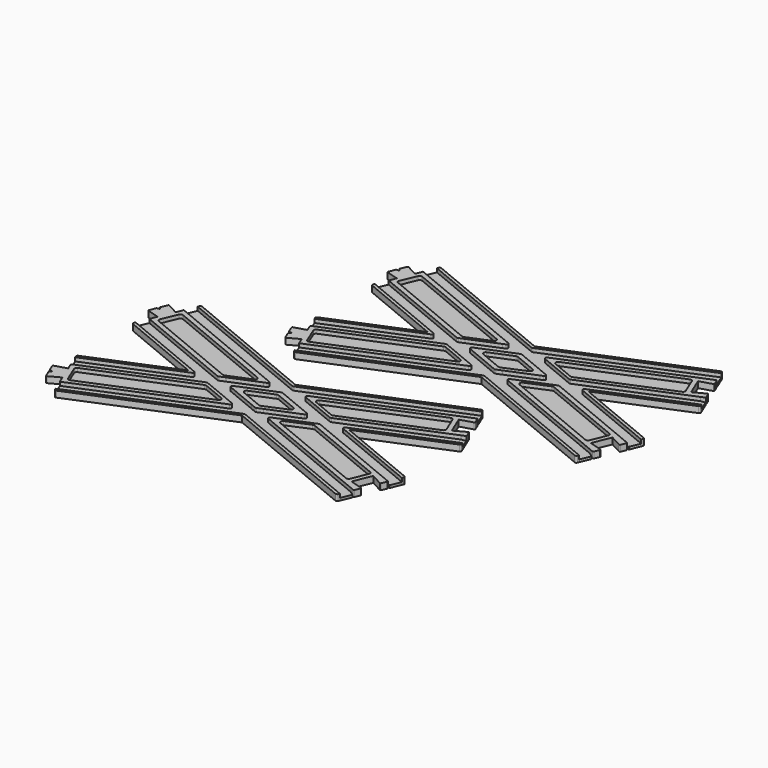
from build123d import *

# Parameters (mm, degrees)
F1_DEPTH = 0.8
F2_DEPTH = 2


# Not quite as in the source:
# - a feature names something its author has since deleted; it is built from what else it names


with BuildPart() as f1:
    # F0 (on Top) → F1 (new body)
    with BuildSketch(Plane.XY):
        with BuildLine():
            Line((-26.799640073, -15.3443313502), (-63.0164195978, -0.3428500855))
            ThreePointArc((-63.0164195978, -0.3428500855), (-63.5904447463, -0.3428500855), (-63.9963418214, -0.7487471607))
            Line((-63.9963418214, -0.7487471607), (-66.1011006995, -5.8300845895))
            ThreePointArc((-66.1011006995, -5.8300845895), (-66.1011006995, -6.404109738), (-65.6952036243, -6.8100068131))
            Line((-65.6952036243, -6.8100068131), (-34.6554323865, -19.6671010328))
            ThreePointArc((-34.6554323865, -19.6671010328), (-34.2727489541, -19.7432215003), (-33.8900655217, -19.6671010328))
            Line((-33.8900655217, -19.6671010328), (-26.799640073, -16.730150649))
            ThreePointArc((-26.799640073, -16.730150649), (-26.3366526473, -16.0372409996), (-26.799640073, -15.3443313502))
        make_face()
    extrude(amount=F1_DEPTH)


with BuildPart() as f1b:
    # F0 (on Top) → F1, piece 2 (new body)
    with BuildSketch(Plane.XY):
        with BuildLine():
            Line((-41.3631744028, -23.7656999509), (-69.878690808, -35.577213584))
            Line((-69.878690808, -35.577213584), (-68.3479570786, -39.272731714))
            Line((-68.3479570786, -39.272731714), (-35.3087138689, -25.587429086))
            ThreePointArc((-35.3087138689, -25.587429086), (-35.0217012946, -25.5303387354), (-34.7346887203, -25.587429086))
            Line((-34.7346887203, -25.587429086), (-23.0712928945, -30.4185658204))
            ThreePointArc((-23.0712928945, -30.4185658204), (-22.7626346107, -30.8805055866), (-23.0712928945, -31.3424453529))
            Line((-23.0712928945, -31.3424453529), (-64.5211227549, -48.5115270391))
            Line((-64.5211227549, -48.5115270391), (-62.9903890255, -52.2070451692))
            Line((-62.9903890255, -52.2070451692), (-17.0168323606, -33.1641744881))
            ThreePointArc((-17.0168323606, -33.1641744881), (-16.7298197863, -33.1070841375), (-16.4428072121, -33.1641744881))
            Line((-16.4428072121, -33.1641744881), (29.5314184974, -52.2073222965))
            Line((29.5314184974, -52.2073222965), (30.9090788598, -48.8813559653))
            Line((30.9090788598, -48.8813559653), (29.6756608657, -47.9375006406))
            Line((29.6756608657, -47.9375006406), (-10.3883466781, -31.3424453529))
            ThreePointArc((-10.3883466781, -31.3424453529), (-10.697004962, -30.8805055866), (-10.3883466781, -30.4185658204))
            Line((-10.3883466781, -30.4185658204), (-9.5437234795, -30.0687114364))
            Line((-9.5437234795, -30.0687114364), (-0.3977827254, -26.2803387354))
            Line((-0.3977827254, -26.2803387354), (1.2750493395, -25.5874290065))
            ThreePointArc((1.2750493395, -25.5874290065), (1.5620619138, -25.5303386559), (1.8490744881, -25.5874290065))
            Line((1.8490744881, -25.5874290065), (33.5024952456, -38.6987051798))
            Line((33.5024952456, -38.6987051798), (35.0420599293, -38.9034570142))
            Line((35.0420599293, -38.9034570142), (36.4197203362, -35.5774905756))
            Line((36.4197203362, -35.5774905756), (7.903535022, -23.7656998714))
            ThreePointArc((7.903535022, -23.7656998714), (7.5948767382, -23.3037601051), (7.903535022, -22.8418203389))
            Line((7.903535022, -22.8418203389), (36.4190482408, -11.0303080256))
            Line((36.4190482408, -11.0303080256), (35.0413878843, -7.7043417086))
            Line((35.0413878843, -7.7043417086), (33.5024956723, -7.9088148537))
            Line((33.5024956723, -7.9088148537), (1.8490744881, -21.0200912037))
            ThreePointArc((1.8490744881, -21.0200912037), (1.5620619138, -21.0771815543), (1.2750493395, -21.0200912037))
            Line((1.2750493395, -21.0200912037), (-10.3883464863, -16.1889544693))
            ThreePointArc((-10.3883464863, -16.1889544693), (-10.6970047701, -15.7270147031), (-10.3883464863, -15.2650749368))
            Line((-10.3883464863, -15.2650749368), (29.6756612258, 1.3299804205))
            Line((29.6756612258, 1.3299804205), (30.9084068147, 2.2735572425))
            Line((30.9084068147, 2.2735572425), (29.5307464582, 5.5995235596))
            Line((29.5307464582, 5.5995235596), (-16.4428070202, -13.4433458017))
            ThreePointArc((-16.4428070202, -13.4433458017), (-16.7298195945, -13.5004361523), (-17.0168321687, -13.4433458017))
            Line((-17.0168321687, -13.4433458017), (-62.9903896117, 5.5995252018))
            Line((-62.9903896117, 5.5995252018), (-64.5211233412, 1.9040070717))
            Line((-64.5211233412, 1.9040070717), (-23.0712927027, -15.2650749368))
            ThreePointArc((-23.0712927027, -15.2650749368), (-22.7626344189, -15.7270147031), (-23.0712927027, -16.1889544693))
            Line((-23.0712927027, -16.1889544693), (-23.9159160932, -16.5388089328))
            Line((-23.9159160932, -16.5388089328), (-33.0618568473, -20.3271816338))
            Line((-33.0618568473, -20.3271816338), (-34.7346887203, -21.0200912832))
            ThreePointArc((-34.7346887203, -21.0200912832), (-35.0217012946, -21.0771816338), (-35.3087138689, -21.0200912832))
            Line((-35.3087138689, -21.0200912832), (-68.347957721, -7.3347883891))
            Line((-68.347957721, -7.3347883891), (-69.8786914505, -11.0303065191))
            Line((-69.8786914505, -11.0303065191), (-41.3631744028, -22.8418204183))
            ThreePointArc((-41.3631744028, -22.8418204183), (-41.054516119, -23.3037601846), (-41.3631744028, -23.7656999509))
        make_face()
        with BuildLine():
            Line((-18.6432387783, -27.9231570891), (-28.6802281864, -23.7656999509))
            ThreePointArc((-28.6802281864, -23.7656999509), (-28.9888864702, -23.3037601846), (-28.6802281864, -22.8418204183))
            Line((-28.6802281864, -22.8418204183), (-27.8356049878, -22.4919660344))
            Line((-27.8356049878, -22.4919660344), (-18.6896642337, -18.7035933334))
            Line((-18.6896642337, -18.7035933334), (-18.6432384455, -18.6843631422))
            Line((-18.6432384455, -18.6843631422), (-17.0168321687, -18.0106836045))
            ThreePointArc((-17.0168321687, -18.0106836045), (-16.7298195945, -17.9535932539), (-16.4428070202, -18.0106836045))
            Line((-16.4428070202, -18.0106836045), (-14.8164043984, -18.6843616283))
            Line((-14.8164043984, -18.6843616283), (-14.7699751472, -18.7035932539))
            Line((-14.7699751472, -18.7035932539), (-4.7794111944, -22.8418203389))
            ThreePointArc((-4.7794111944, -22.8418203389), (-4.4707529106, -23.3037601051), (-4.7794111944, -23.7656998714))
            Line((-4.7794111944, -23.7656998714), (-5.6240345849, -24.1155543348))
            Line((-5.6240345849, -24.1155543348), (-14.769975339, -27.9039270358))
            Line((-14.769975339, -27.9039270358), (-16.4428072121, -28.5968366852))
            ThreePointArc((-16.4428072121, -28.5968366852), (-16.7298197863, -28.6539270358), (-17.0168323606, -28.5968366852))
            Line((-17.0168323606, -28.5968366852), (-18.6432387783, -27.9231570891))
        make_face(mode=Mode.SUBTRACT)
    extrude(amount=F1_DEPTH)


with BuildPart() as f1c:
    # F0 (on Top) → F1, piece 3 (new body)
    with BuildSketch(Plane.XY):
        with BuildLine():
            Line((-34.7511032445, -26.9800475033), (-65.6952029819, -39.79751329))
            ThreePointArc((-65.6952029819, -39.79751329), (-66.101100057, -40.2034103651), (-66.101100057, -40.7774355136))
            Line((-66.101100057, -40.7774355136), (-63.996341179, -45.8587729424))
            ThreePointArc((-63.996341179, -45.8587729424), (-63.5904441039, -46.2646700175), (-63.0164189553, -46.2646700175))
            Line((-63.0164189553, -46.2646700175), (-26.8953109311, -31.302817186))
            ThreePointArc((-26.8953109311, -31.302817186), (-26.4323235054, -30.6099075366), (-26.8953109311, -29.9169978872))
            Line((-26.8953109311, -29.9169978872), (-33.9857363798, -26.9800475033))
            ThreePointArc((-33.9857363798, -26.9800475033), (-34.3684198122, -26.9039270358), (-34.7511032445, -26.9800475033))
        make_face()
    extrude(amount=F1_DEPTH)


with BuildPart() as f1d:
    # F0 (on Top) → F1, piece 4 (new body)
    with BuildSketch(Plane.XY):
        with BuildLine():
            ThreePointArc((-24.2029286674, -22.6108505352), (-24.6659160932, -23.3037601846), (-24.2029286674, -23.996669834))
            Line((-24.2029286674, -23.996669834), (-17.0168323606, -26.9732483848))
            ThreePointArc((-17.0168323606, -26.9732483848), (-16.629331896, -27.0493572503), (-16.2425826435, -26.9695187556))
            Line((-16.2425826435, -26.9695187556), (-9.250048766, -23.9938726121))
            ThreePointArc((-9.250048766, -23.9938726121), (-8.793732181, -23.3001474104), (-9.2567109053, -22.6108505352))
            Line((-9.2567109053, -22.6108505352), (-16.347136354, -19.6739001514))
            ThreePointArc((-16.347136354, -19.6739001514), (-16.7298197863, -19.5977796839), (-17.1125032187, -19.6739001514))
            Line((-17.1125032187, -19.6739001514), (-24.2029286674, -22.6108505352))
        make_face()
    extrude(amount=F1_DEPTH)


with BuildPart() as f1e:
    # F0 (on Top) → F1, piece 5 (new body)
    with BuildSketch(Plane.XY):
        with BuildLine():
            Line((28.532860387, -7.6111790722), (26.4000801634, -2.4621921308))
            ThreePointArc((26.4000801634, -2.4621921308), (25.9941830883, -2.0562950557), (25.4201579397, -2.0562950557))
            Line((25.4201579397, -2.0562950557), (-6.5643284497, -15.3047031038))
            ThreePointArc((-6.5643284497, -15.3047031038), (-7.0273158755, -15.9976127532), (-6.5643284497, -16.6905224025))
            Line((-6.5643284497, -16.6905224025), (0.6217678571, -19.6671009533))
            ThreePointArc((0.6217678571, -19.6671009533), (1.0044512894, -19.7432214208), (1.3871347218, -19.6671009533))
            Line((1.3871347218, -19.6671009533), (28.1269633119, -8.5911012958))
            ThreePointArc((28.1269633119, -8.5911012958), (28.532860387, -8.1852042207), (28.532860387, -7.6111790722))
        make_face()
    extrude(amount=F1_DEPTH)


with BuildPart() as f1f:
    # F0 (on Top) → F1, piece 6 (new body)
    with BuildSketch(Plane.XY):
        with BuildLine():
            Line((26.4000800865, -44.1453282065), (28.5048389645, -39.0639907777))
            ThreePointArc((28.5048389645, -39.0639907777), (28.5048389645, -38.4899656292), (28.0989418894, -38.0840685541))
            Line((28.0989418894, -38.0840685541), (1.1957928138, -26.9404193364))
            ThreePointArc((1.1957928138, -26.9404193364), (0.8082923491, -26.8643104709), (0.4215430966, -26.9441489655))
            Line((0.4215430966, -26.9441489655), (-6.5709907809, -29.9197951091))
            ThreePointArc((-6.5709907809, -29.9197951091), (-7.0273073659, -30.6135203108), (-6.5643286416, -31.302817186))
            Line((-6.5643286416, -31.302817186), (25.4201578629, -44.5512252817))
            ThreePointArc((25.4201578629, -44.5512252817), (25.9941830114, -44.5512252817), (26.4000800865, -44.1453282065))
        make_face()
    extrude(amount=F1_DEPTH)


with BuildPart() as f1g:
    # F0 (on Top) → F1, piece 7 (new body)
    with BuildSketch(Plane.XY):
        with BuildLine():
            Line((-7.114914129, 30.7077025481), (-35.6304305342, 18.896188915))
            Line((-35.6304305342, 18.896188915), (-34.0996968047, 15.200670785))
            Line((-34.0996968047, 15.200670785), (-1.060453595, 28.885973413))
            ThreePointArc((-1.060453595, 28.885973413), (-0.7734410208, 28.9430637636), (-0.4864284465, 28.885973413))
            Line((-0.4864284465, 28.885973413), (11.1769673793, 24.0548366786))
            ThreePointArc((11.1769673793, 24.0548366786), (11.4856256631, 23.5928969123), (11.1769673793, 23.1309571461))
            Line((11.1769673793, 23.1309571461), (-30.2728624811, 5.9618754599))
            Line((-30.2728624811, 5.9618754598), (-28.7421287516, 2.2663573298))
            Line((-28.7421287516, 2.2663573298), (17.2314279132, 21.3092280109))
            ThreePointArc((17.2314279132, 21.3092280109), (17.5184404875, 21.3663183615), (17.8054530618, 21.3092280109))
            Line((17.8054530618, 21.3092280109), (63.7796787572, 2.2660802083))
            Line((63.7796787572, 2.2660802083), (65.1573391196, 5.5920465395))
            Line((65.1573391196, 5.5920465395), (63.9239211396, 6.5359018584))
            Line((63.9239211396, 6.5359018584), (23.8599135957, 23.1309571461))
            ThreePointArc((23.8599135957, 23.1309571461), (23.5512553119, 23.5928969123), (23.8599135957, 24.0548366786))
            Line((23.8599135957, 24.0548366786), (24.7045367943, 24.4046910626))
            Line((24.7045367943, 24.4046910626), (33.8504775485, 28.1930637636))
            Line((33.8504775485, 28.1930637636), (35.5233096134, 28.8859734924))
            ThreePointArc((35.5233096134, 28.8859734924), (35.8103221876, 28.9430638431), (36.0973347619, 28.8859734924))
            Line((36.0973347619, 28.8859734924), (67.7507555194, 15.7746973192))
            Line((67.7507555194, 15.7746973192), (69.2903201891, 15.5699454906))
            Line((69.2903201891, 15.5699454906), (70.667980596, 18.8959119292))
            Line((70.667980596, 18.8959119292), (42.1517952958, 30.7077026276))
            ThreePointArc((42.1517952958, 30.7077026276), (41.843137012, 31.1696423939), (42.1517952958, 31.6315821601))
            Line((42.1517952958, 31.6315821601), (70.6673085146, 43.4430944734))
            Line((70.6673085146, 43.4430944734), (69.2896481581, 46.7690607904))
            Line((69.2896481581, 46.7690607904), (67.7507559462, 46.5645876453))
            Line((67.7507559462, 46.5645876453), (36.0973347619, 33.4533112953))
            ThreePointArc((36.0973347619, 33.4533112953), (35.8103221876, 33.3962209447), (35.5233096134, 33.4533112953))
            Line((35.5233096134, 33.4533112953), (23.8599137876, 38.2844480297))
            ThreePointArc((23.8599137876, 38.2844480297), (23.5512555037, 38.7463877959), (23.8599137876, 39.2083275622))
            Line((23.8599137876, 39.2083275622), (63.9239214996, 55.8033829195))
            Line((63.9239214996, 55.8033829195), (65.1566670886, 56.7469597415))
            Line((65.1566670886, 56.7469597415), (63.7790067321, 60.0729260586))
            Line((63.7790067321, 60.0729260586), (17.8054532536, 41.0300566973))
            ThreePointArc((17.8054532536, 41.0300566973), (17.5184406794, 40.9729663467), (17.2314281051, 41.0300566973))
            Line((17.2314281051, 41.0300566973), (-28.7421293379, 60.0729277008))
            Line((-28.7421293379, 60.0729277008), (-30.2728630674, 56.3774095707))
            Line((-30.2728630674, 56.3774095707), (11.1769675712, 39.2083275622))
            ThreePointArc((11.1769675712, 39.2083275622), (11.485625855, 38.7463877959), (11.1769675712, 38.2844480297))
            Line((11.1769675712, 38.2844480297), (10.3323441807, 37.9345935662))
            Line((10.3323441807, 37.9345935662), (1.1864034265, 34.1462208652))
            Line((1.1864034265, 34.1462208652), (-0.4864284465, 33.4533112158))
            ThreePointArc((-0.4864284465, 33.4533112158), (-0.7734410208, 33.3962208652), (-1.060453595, 33.4533112158))
            Line((-1.060453595, 33.4533112158), (-34.0996974472, 47.1386141099))
            Line((-34.0996974472, 47.1386141099), (-35.6304311767, 43.4430959799))
            Line((-35.6304311767, 43.4430959799), (-7.114914129, 31.6315820806))
            ThreePointArc((-7.114914129, 31.6315820806), (-6.8062558452, 31.1696423144), (-7.114914129, 30.7077025481))
        make_face()
        with BuildLine():
            Line((15.6050214956, 26.5502454099), (5.5680320874, 30.7077025481))
            ThreePointArc((5.5680320874, 30.7077025481), (5.2593738036, 31.1696423144), (5.5680320874, 31.6315820806))
            Line((5.5680320874, 31.6315820806), (6.412655286, 31.9814364646))
            Line((6.412655286, 31.9814364646), (15.5585960402, 35.7698091656))
            Line((15.5585960402, 35.7698091656), (15.6050218284, 35.7890393567))
            Line((15.6050218284, 35.7890393567), (17.2314281051, 36.4627188945))
            ThreePointArc((17.2314281051, 36.4627188945), (17.5184406794, 36.5198092451), (17.8054532536, 36.4627188945))
            Line((17.8054532536, 36.4627188945), (19.4318558754, 35.7890408707))
            Line((19.4318558754, 35.7890408707), (19.4782851267, 35.7698092451))
            Line((19.4782851267, 35.7698092451), (29.4688490794, 31.6315821601))
            ThreePointArc((29.4688490794, 31.6315821601), (29.7775073633, 31.1696423939), (29.4688490794, 30.7077026276))
            Line((29.4688490794, 30.7077026276), (28.6242256889, 30.3578481642))
            Line((28.6242256889, 30.3578481642), (19.4782849348, 26.5694754631))
            Line((19.4782849348, 26.5694754631), (17.8054530618, 25.8765658138))
            ThreePointArc((17.8054530618, 25.8765658138), (17.5184404875, 25.8194754631), (17.2314279132, 25.8765658138))
            Line((17.2314279132, 25.8765658138), (15.6050214956, 26.5502454099))
        make_face(mode=Mode.SUBTRACT)
    extrude(amount=F1_DEPTH)


with BuildPart() as f1h:
    # F0 (on Top) → F1, piece 8 (new body)
    with BuildSketch(Plane.XY):
        with BuildLine():
            Line((7.4486202008, 39.1290711488), (-28.768159324, 54.1305524134))
            ThreePointArc((-28.768159324, 54.1305524134), (-29.3421844725, 54.1305524134), (-29.7480815476, 53.7246553383))
            Line((-29.7480815476, 53.7246553383), (-31.8528404256, 48.6433179095))
            ThreePointArc((-31.8528404256, 48.6433179095), (-31.8528404256, 48.069292761), (-31.4469433505, 47.6633956859))
            Line((-31.4469433505, 47.6633956859), (-0.4071721126, 34.8063014662))
            ThreePointArc((-0.4071721126, 34.8063014662), (-0.0244886802, 34.7301809987), (0.3581947521, 34.8063014662))
            Line((0.3581947521, 34.8063014662), (7.4486202008, 37.74325185))
            ThreePointArc((7.4486202008, 37.74325185), (7.9116076266, 38.4361614994), (7.4486202008, 39.1290711488))
        make_face()
    extrude(amount=F1_DEPTH)


with BuildPart() as f1i:
    # F0 (on Top) → F1, piece 9 (new body)
    with BuildSketch(Plane.XY):
        with BuildLine():
            ThreePointArc((10.0453316064, 31.8625519638), (9.5823441807, 31.1696423144), (10.0453316064, 30.476732665))
            Line((10.0453316064, 30.476732665), (17.2314279132, 27.5001541142))
            ThreePointArc((17.2314279132, 27.5001541142), (17.6189283779, 27.4240452487), (18.0056776303, 27.5038837433))
            Line((18.0056776303, 27.5038837433), (24.9982115079, 30.4795298869))
            ThreePointArc((24.9982115079, 30.4795298869), (25.4545280928, 31.1732550886), (24.9915493686, 31.8625519638))
            Line((24.9915493686, 31.8625519638), (17.9011239199, 34.7995023476))
            ThreePointArc((17.9011239199, 34.7995023476), (17.5184404875, 34.8756228151), (17.1357570551, 34.7995023476))
            Line((17.1357570551, 34.7995023476), (10.0453316064, 31.8625519638))
        make_face()
    extrude(amount=F1_DEPTH)


with BuildPart() as f1j:
    # F0 (on Top) → F1, piece 10 (new body)
    with BuildSketch(Plane.XY):
        with BuildLine():
            Line((62.7811206608, 46.8622234268), (60.6483404372, 52.0112103682))
            ThreePointArc((60.6483404372, 52.0112103682), (60.2424433621, 52.4171074433), (59.6684182136, 52.4171074433))
            Line((59.6684182136, 52.4171074433), (27.6839318241, 39.1686993952))
            ThreePointArc((27.6839318241, 39.1686993952), (27.2209443984, 38.4757897458), (27.6839318241, 37.7828800964))
            Line((27.6839318241, 37.7828800964), (34.8700281309, 34.8063015456))
            ThreePointArc((34.8700281309, 34.8063015456), (35.2527115633, 34.7301810782), (35.6353949957, 34.8063015456))
            Line((35.6353949957, 34.8063015456), (62.3752235857, 45.8823012032))
            ThreePointArc((62.3752235857, 45.8823012032), (62.7811206608, 46.2881982783), (62.7811206608, 46.8622234268))
        make_face()
    extrude(amount=F1_DEPTH)


with BuildPart() as f1k:
    # F0 (on Top) → F1, piece 11 (new body)
    with BuildSketch(Plane.XY):
        with BuildLine():
            Line((60.6483403619, 10.3280742918), (62.7530992399, 15.4094117206))
            ThreePointArc((62.7530992399, 15.4094117206), (62.7530992399, 15.9834368692), (62.3472021648, 16.3893339443))
            Line((62.3472021648, 16.3893339443), (35.4440530876, 27.5329831626))
            ThreePointArc((35.4440530876, 27.5329831626), (35.0565526229, 27.6090920281), (34.6698033705, 27.5292535334))
            Line((34.6698033705, 27.5292535334), (27.6772694929, 24.5536073899))
            ThreePointArc((27.6772694929, 24.5536073899), (27.220952908, 23.8598821882), (27.6839316322, 23.170585313))
            Line((27.6839316322, 23.170585313), (59.6684181383, 9.9221772167))
            ThreePointArc((59.6684181383, 9.9221772167), (60.2424432868, 9.9221772167), (60.6483403619, 10.3280742918))
        make_face()
    extrude(amount=F1_DEPTH)


with BuildPart() as f1l:
    # F0 (on Top) → F1, piece 12 (new body)
    with BuildSketch(Plane.XY):
        with BuildLine():
            Line((-0.5028429707, 27.4933549957), (-31.446942708, 14.675889209))
            ThreePointArc((-31.446942708, 14.675889209), (-31.8528397832, 14.2699921339), (-31.8528397832, 13.6959669854))
            Line((-31.8528397832, 13.6959669854), (-29.7480809051, 8.6146295565))
            ThreePointArc((-29.7480809051, 8.6146295565), (-29.34218383, 8.2087324814), (-28.7681586815, 8.2087324814))
            Line((-28.7681586815, 8.2087324814), (7.3529493428, 23.170585313))
            ThreePointArc((7.3529493428, 23.170585313), (7.8159367685, 23.8634949624), (7.3529493428, 24.5564046118))
            Line((7.3529493428, 24.5564046118), (0.262523894, 27.4933549957))
            ThreePointArc((0.262523894, 27.4933549957), (-0.1201595383, 27.5694754631), (-0.5028429707, 27.4933549957))
        make_face()
    extrude(amount=F1_DEPTH)


with BuildPart() as f2:
    # F0 (on Top) → F2 (new body)
    with BuildSketch(Plane.XY):
        with BuildLine():
            Line((-67.4295174834, -5.117477511), (-68.347957721, -7.3347883891))
            Line((-68.347957721, -7.3347883891), (-35.3087138689, -21.0200912832))
            ThreePointArc((-35.3087138689, -21.0200912832), (-35.0217012946, -21.0771816338), (-34.7346887203, -21.0200912832))
            Line((-34.7346887203, -21.0200912832), (-33.0618568473, -20.3271816338))
            Line((-33.0618568473, -20.3271816338), (-23.9159160932, -16.5388089328))
            Line((-23.9159160932, -16.5388089328), (-23.0712927027, -16.1889544693))
            ThreePointArc((-23.0712927027, -16.1889544693), (-22.7626344189, -15.7270147031), (-23.0712927027, -15.2650749368))
            Line((-23.0712927027, -15.2650749368), (-64.5211233412, 1.9040070717))
            Line((-64.5211233412, 1.9040070717), (-65.4395635789, -0.3133038063))
            Line((-65.4395635789, -0.3133038063), (-68.9742038238, 1.6064137918))
            ThreePointArc((-68.9742038238, 1.6064137918), (-69.1769577929, 1.6223897475), (-69.3244904948, 1.4823950868))
            Line((-69.3244904948, 1.4823950868), (-70.1940668164, -0.6169478625))
            Line((-70.1940668164, -0.6169478625), (-69.5853053874, -1.4103012028))
            Line((-69.5853053874, -1.4103012028), (-70.5767502345, -1.5408274009))
            Line((-70.5767502345, -1.5408274009), (-71.4463265525, -3.6401703414))
            ThreePointArc((-71.4463265525, -3.6401703414), (-71.4409963507, -3.8434828932), (-71.2863309312, -3.9755548915))
            Line((-71.2863309312, -3.9755548915), (-67.4295174834, -5.117477511))
        make_face()
        with BuildLine():
            ThreePointArc((-63.9963418214, -0.7487471607), (-63.5904447463, -0.3428500855), (-63.0164195978, -0.3428500855))
            Line((-63.0164195978, -0.3428500855), (-26.799640073, -15.3443313502))
            ThreePointArc((-26.799640073, -15.3443313502), (-26.3366526473, -16.0372409996), (-26.799640073, -16.730150649))
            Line((-26.799640073, -16.730150649), (-33.8900655217, -19.6671010328))
            ThreePointArc((-33.8900655217, -19.6671010328), (-34.2727489541, -19.7432215003), (-34.6554323865, -19.6671010328))
            Line((-34.6554323865, -19.6671010328), (-65.6952036243, -6.8100068131))
            ThreePointArc((-65.6952036243, -6.8100068131), (-66.1011006995, -6.404109738), (-66.1011006995, -5.8300845895))
            Line((-66.1011006995, -5.8300845895), (-63.9963418214, -0.7487471607))
        make_face(mode=Mode.SUBTRACT)
    extrude(amount=F2_DEPTH)


with BuildPart() as f2b:
    # F0 (on Top) → F2, piece 2 (new body)
    with BuildSketch(Plane.XY):
        with BuildLine():
            Line((-42.8610790839, -23.3037601846), (-69.7994344742, -34.4619923353))
            ThreePointArc((-69.7994344742, -34.4619923353), (-70.0700325242, -34.7325903854), (-70.0700325242, -35.1152738177))
            Line((-70.0700325242, -35.1152738177), (-69.878690808, -35.577213584))
            Line((-69.878690808, -35.577213584), (-41.3631744028, -23.7656999509))
            ThreePointArc((-41.3631744028, -23.7656999509), (-41.054516119, -23.3037601846), (-41.3631744028, -22.8418204183))
            Line((-41.3631744028, -22.8418204183), (-69.8786914505, -11.0303065191))
            Line((-69.8786914505, -11.0303065191), (-70.0700331667, -11.4922462854))
            ThreePointArc((-70.0700331667, -11.4922462854), (-70.0700331667, -11.8749297177), (-69.7994351166, -12.1455277678))
            Line((-69.7994351166, -12.1455277678), (-42.8610790839, -23.3037601846))
        make_face()
    extrude(amount=F2_DEPTH)


with BuildPart() as f2c:
    # F0 (on Top) → F2, piece 3 (new body)
    with BuildSketch(Plane.XY):
        with BuildLine():
            Line((-35.3087138689, -25.587429086), (-68.3479570786, -39.272731714))
            Line((-68.3479570786, -39.272731714), (-67.4295168409, -41.490042592))
            Line((-67.4295168409, -41.490042592), (-71.2863302887, -42.6319652115))
            ThreePointArc((-71.2863302887, -42.6319652115), (-71.4409957082, -42.7640372099), (-71.4463259101, -42.9673497617))
            Line((-71.4463259101, -42.9673497617), (-70.5767495921, -45.0666927021))
            Line((-70.5767495921, -45.0666927021), (-69.5853047307, -45.1972188944))
            Line((-69.5853047307, -45.1972188944), (-70.1940661597, -45.9905722347))
            Line((-70.1940661597, -45.9905722347), (-69.3244898417, -48.0899151751))
            ThreePointArc((-69.3244898417, -48.0899151751), (-69.1769571358, -48.2299098373), (-68.9742031631, -48.213933876))
            Line((-68.9742031631, -48.213933876), (-65.4395629926, -46.2942161611))
            Line((-65.4395629926, -46.2942161611), (-64.5211227549, -48.5115270391))
            Line((-64.5211227549, -48.5115270391), (-23.0712928945, -31.3424453529))
            ThreePointArc((-23.0712928945, -31.3424453529), (-22.7626346107, -30.8805055866), (-23.0712928945, -30.4185658204))
            Line((-23.0712928945, -30.4185658204), (-34.7346887203, -25.587429086))
            ThreePointArc((-34.7346887203, -25.587429086), (-35.0217012946, -25.5303387354), (-35.3087138689, -25.587429086))
        make_face()
        with BuildLine():
            ThreePointArc((-66.101100057, -40.7774355136), (-66.101100057, -40.2034103651), (-65.6952029819, -39.79751329))
            Line((-65.6952029819, -39.79751329), (-34.7511032445, -26.9800475033))
            ThreePointArc((-34.7511032445, -26.9800475033), (-34.3684198122, -26.9039270358), (-33.9857363798, -26.9800475033))
            Line((-33.9857363798, -26.9800475033), (-26.8953109311, -29.9169978872))
            ThreePointArc((-26.8953109311, -29.9169978872), (-26.4323235054, -30.6099075366), (-26.8953109311, -31.302817186))
            Line((-26.8953109311, -31.302817186), (-63.0164189553, -46.2646700175))
            ThreePointArc((-63.0164189553, -46.2646700175), (-63.5904441039, -46.2646700175), (-63.996341179, -45.8587729424))
            Line((-63.996341179, -45.8587729424), (-66.101100057, -40.7774355136))
        make_face(mode=Mode.SUBTRACT)
    extrude(amount=F2_DEPTH)


with BuildPart() as f2d:
    # F0 (on Top) → F2, piece 4 (new body)
    with BuildSketch(Plane.XY):
        with BuildLine():
            Line((-17.0168323606, -33.1641744881), (-62.9903890255, -52.2070451692))
            Line((-62.9903890255, -52.2070451692), (-62.7990473093, -52.6689849354))
            ThreePointArc((-62.7990473093, -52.6689849354), (-62.5284492592, -52.9395829855), (-62.1457658269, -52.9395829855))
            Line((-62.1457658269, -52.9395829855), (-16.7298197863, -34.1276821875))
            Line((-16.7298197863, -34.1276821875), (28.6867952988, -52.9398601129))
            ThreePointArc((28.6867952988, -52.9398601129), (29.0694787311, -52.9398601129), (29.3400767812, -52.6692620628))
            Line((29.3400767812, -52.6692620628), (29.5314184974, -52.2073222965))
            Line((29.5314184974, -52.2073222965), (-16.4428072121, -33.1641744881))
            ThreePointArc((-16.4428072121, -33.1641744881), (-16.7298197863, -33.1070841375), (-17.0168323606, -33.1641744881))
        make_face()
    extrude(amount=F2_DEPTH)


with BuildPart() as f2e:
    # F0 (on Top) → F2, piece 5 (new body)
    with BuildSketch(Plane.XY):
        with BuildLine():
            Line((-10.3883466781, -31.3424453529), (29.6756608657, -47.9375006406))
            Line((29.6756608657, -47.9375006406), (30.8311092685, -48.4161030396))
            ThreePointArc((30.8311092685, -48.4161030396), (31.0224875153, -48.4160879048), (31.1577802621, -48.2807309461))
            Line((31.1577802621, -48.2807309461), (31.8359982031, -46.6419018804))
            ThreePointArc((31.8359982031, -46.6419018804), (31.8308718378, -46.4391544761), (31.6770923803, -46.3069248726))
            Line((31.6770923803, -46.3069248726), (27.6328260153, -45.0889051693))
            Line((27.6328260153, -45.0889051693), (30.0437317475, -39.2684640004))
            Line((30.0437317475, -39.2684640004), (33.764729932, -41.2669221325))
            ThreePointArc((33.764729932, -41.2669221325), (33.9669688804, -41.2821601773), (34.1139578305, -41.142420996))
            Line((34.1139578305, -41.142420996), (34.7932124067, -39.5040213753))
            ThreePointArc((34.7932124067, -39.5040213753), (34.7932578074, -39.3126431364), (34.6579436546, -39.1773075814))
            Line((34.6579436546, -39.1773075814), (33.5024952456, -38.6987051798))
            Line((33.5024952456, -38.6987051798), (1.8490744881, -25.5874290065))
            ThreePointArc((1.8490744881, -25.5874290065), (1.5620619138, -25.5303386559), (1.2750493395, -25.5874290065))
            Line((1.2750493395, -25.5874290065), (-0.3977827254, -26.2803387354))
            Line((-0.3977827254, -26.2803387354), (-9.5437234795, -30.0687114364))
            Line((-9.5437234795, -30.0687114364), (-10.3883466781, -30.4185658204))
            ThreePointArc((-10.3883466781, -30.4185658204), (-10.697004962, -30.8805055866), (-10.3883466781, -31.3424453529))
        make_face()
        with BuildLine():
            ThreePointArc((28.0989418894, -38.0840685541), (28.5048389645, -38.4899656292), (28.5048389645, -39.0639907777))
            Line((28.5048389645, -39.0639907777), (26.4000800865, -44.1453282065))
            ThreePointArc((26.4000800865, -44.1453282065), (25.9941830114, -44.5512252817), (25.4201578629, -44.5512252817))
            Line((25.4201578629, -44.5512252817), (-6.5643286416, -31.302817186))
            ThreePointArc((-6.5643286416, -31.302817186), (-7.0273073659, -30.6135203108), (-6.5709907809, -29.9197951091))
            Line((-6.5709907809, -29.9197951091), (0.4215430966, -26.9441489655))
            ThreePointArc((0.4215430966, -26.9441489655), (0.8082923491, -26.8643104709), (1.1957928138, -26.9404193364))
            Line((1.1957928138, -26.9404193364), (28.0989418894, -38.0840685541))
        make_face(mode=Mode.SUBTRACT)
    extrude(amount=F2_DEPTH)


with BuildPart() as f2f:
    # F0 (on Top) → F2, piece 6 (new body)
    with BuildSketch(Plane.XY):
        with BuildLine():
            Line((7.903535022, -23.7656998714), (36.4197203362, -35.5774905756))
            Line((36.4197203362, -35.5774905756), (36.6110620523, -35.1155508094))
            ThreePointArc((36.6110620523, -35.1155508094), (36.6110620523, -34.732867377), (36.3404640023, -34.462269327))
            Line((36.3404640023, -34.462269327), (9.4014397031, -23.3037601051))
            Line((9.4014397031, -23.3037601051), (36.3397919069, -12.1455292743))
            ThreePointArc((36.3397919069, -12.1455292743), (36.610389957, -11.8749312242), (36.610389957, -11.4922477919))
            Line((36.610389957, -11.4922477919), (36.4190482408, -11.0303080256))
            Line((36.4190482408, -11.0303080256), (7.903535022, -22.8418203389))
            ThreePointArc((7.903535022, -22.8418203389), (7.5948767382, -23.3037601051), (7.903535022, -23.7656998714))
        make_face()
    extrude(amount=F2_DEPTH)


with BuildPart() as f2g:
    # F0 (on Top) → F2, piece 7 (new body)
    with BuildSketch(Plane.XY):
        with BuildLine():
            Line((30.8305103573, 1.8083345933), (29.6756612258, 1.3299804205))
            Line((29.6756612258, 1.3299804205), (-10.3883464863, -15.2650749368))
            ThreePointArc((-10.3883464863, -15.2650749368), (-10.6970047701, -15.7270147031), (-10.3883464863, -16.1889544693))
            Line((-10.3883464863, -16.1889544693), (1.2750493395, -21.0200912037))
            ThreePointArc((1.2750493395, -21.0200912037), (1.5620619138, -21.0771815543), (1.8490744881, -21.0200912037))
            Line((1.8490744881, -21.0200912037), (33.5024956723, -7.9088148537))
            Line((33.5024956723, -7.9088148537), (34.8883145113, -7.3347898956))
            Line((34.8883145113, -7.3347898956), (34.1139106964, -5.465213793))
            ThreePointArc((34.1139106964, -5.465213793), (33.9669287134, -5.3254148419), (33.7646525247, -5.3406396088))
            Line((33.7646525247, -5.3406396088), (30.0437317481, -7.3390562096))
            Line((30.0437317481, -7.3390562096), (27.6328266453, -1.5186149389))
            Line((27.6328266453, -1.5186149389), (31.6770088236, -0.3006205752))
            ThreePointArc((31.6770088236, -0.3006205752), (31.8308052373, -0.1683552187), (31.8358843713, 0.0344295534))
            Line((31.8358843713, 0.0344295534), (31.1571510766, 1.673035621))
            ThreePointArc((31.1571510766, 1.673035621), (31.0218520471, 1.8083346042), (30.8305103573, 1.8083345933))
        make_face()
        with BuildLine():
            ThreePointArc((25.4201579397, -2.0562950557), (25.9941830883, -2.0562950557), (26.4000801634, -2.4621921308))
            Line((26.4000801634, -2.4621921308), (28.532860387, -7.6111790722))
            ThreePointArc((28.532860387, -7.6111790722), (28.532860387, -8.1852042207), (28.1269633119, -8.5911012958))
            Line((28.1269633119, -8.5911012958), (1.3871347218, -19.6671009533))
            ThreePointArc((1.3871347218, -19.6671009533), (1.0044512894, -19.7432214208), (0.6217678571, -19.6671009533))
            Line((0.6217678571, -19.6671009533), (-6.5643284497, -16.6905224025))
            ThreePointArc((-6.5643284497, -16.6905224025), (-7.0273158755, -15.9976127532), (-6.5643284497, -15.3047031038))
            Line((-6.5643284497, -15.3047031038), (25.4201579397, -2.0562950557))
        make_face(mode=Mode.SUBTRACT)
    extrude(amount=F2_DEPTH)


with BuildPart() as f2h:
    # F0 (on Top) → F2, piece 8 (new body)
    with BuildSketch(Plane.XY):
        with BuildLine():
            ThreePointArc((-28.6802281864, -22.8418204183), (-28.9888864702, -23.3037601846), (-28.6802281864, -23.7656999509))
            Line((-28.6802281864, -23.7656999509), (-18.6432387783, -27.9231570891))
            Line((-18.6432387783, -27.9231570891), (-17.0168323606, -28.5968366852))
            ThreePointArc((-17.0168323606, -28.5968366852), (-16.7298197863, -28.6539270358), (-16.4428072121, -28.5968366852))
            Line((-16.4428072121, -28.5968366852), (-14.769975339, -27.9039270358))
            Line((-14.769975339, -27.9039270358), (-5.6240345849, -24.1155543348))
            Line((-5.6240345849, -24.1155543348), (-4.7794111944, -23.7656998714))
            ThreePointArc((-4.7794111944, -23.7656998714), (-4.4707529106, -23.3037601051), (-4.7794111944, -22.8418203389))
            Line((-4.7794111944, -22.8418203389), (-14.7699751472, -18.7035932539))
            Line((-14.7699751472, -18.7035932539), (-14.835636024, -18.7307908796))
            Line((-14.835636024, -18.7307908796), (-14.8164043984, -18.6843616283))
            Line((-14.8164043984, -18.6843616283), (-16.4428070202, -18.0106836045))
            ThreePointArc((-16.4428070202, -18.0106836045), (-16.7298195945, -17.9535932539), (-17.0168321687, -18.0106836045))
            Line((-17.0168321687, -18.0106836045), (-18.6432384455, -18.6843631422))
            Line((-18.6432384455, -18.6843631422), (-18.6896642337, -18.7035933334))
            Line((-18.6896642337, -18.7035933334), (-27.8356049878, -22.4919660344))
            Line((-27.8356049878, -22.4919660344), (-28.6802281864, -22.8418204183))
        make_face()
        with BuildLine():
            Line((-17.0168323606, -26.9732483848), (-24.2029286674, -23.996669834))
            ThreePointArc((-24.2029286674, -23.996669834), (-24.6659160932, -23.3037601846), (-24.2029286674, -22.6108505352))
            Line((-24.2029286674, -22.6108505352), (-17.1125032187, -19.6739001514))
            ThreePointArc((-17.1125032187, -19.6739001514), (-16.7298197863, -19.5977796839), (-16.347136354, -19.6739001514))
            Line((-16.347136354, -19.6739001514), (-9.2567109053, -22.6108505352))
            ThreePointArc((-9.2567109053, -22.6108505352), (-8.793732181, -23.3001474104), (-9.250048766, -23.9938726121))
            Line((-9.250048766, -23.9938726121), (-16.2425826435, -26.9695187556))
            ThreePointArc((-16.2425826435, -26.9695187556), (-16.629331896, -27.0493572503), (-17.0168323606, -26.9732483848))
        make_face(mode=Mode.SUBTRACT)
    extrude(amount=F2_DEPTH)


with BuildPart() as f2i:
    # F0 (on Top) → F2, piece 9 (new body)
    with BuildSketch(Plane.XY):
        with BuildLine():
            Line((-62.7990478956, 6.061464968), (-62.9903896117, 5.5995252018))
            Line((-62.9903896117, 5.5995252018), (-17.0168321687, -13.4433458017))
            ThreePointArc((-17.0168321687, -13.4433458017), (-16.7298195945, -13.5004361523), (-16.4428070202, -13.4433458017))
            Line((-16.4428070202, -13.4433458017), (29.5307464582, 5.5995235596))
            Line((29.5307464582, 5.5995235596), (29.339404742, 6.0614633258))
            ThreePointArc((29.339404742, 6.0614633258), (29.068806692, 6.3320613759), (28.6861232596, 6.3320613759))
            Line((28.6861232596, 6.3320613759), (-16.7298195945, -12.4798381022))
            Line((-16.7298195945, -12.4798381022), (-62.1457664131, 6.3320630181))
            ThreePointArc((-62.1457664131, 6.3320630181), (-62.5284498455, 6.3320630181), (-62.7990478956, 6.061464968))
        make_face()
    extrude(amount=F2_DEPTH)


with BuildPart() as f2j:
    # F0 (on Top) → F2, piece 10 (new body)
    with BuildSketch(Plane.XY):
        with BuildLine():
            Line((-1.060453595, 28.885973413), (-34.0996968047, 15.200670785))
            Line((-34.0996968047, 15.200670785), (-33.1812565671, 12.9833599069))
            Line((-33.1812565671, 12.9833599069), (-37.0380700149, 11.8414372874))
            ThreePointArc((-37.0380700149, 11.8414372874), (-37.1927354344, 11.7093652891), (-37.1980656362, 11.5060527373))
            Line((-37.1980656362, 11.5060527373), (-36.3284893182, 9.4067097968))
            Line((-36.3284893182, 9.4067097968), (-35.3370444569, 9.2761836046))
            Line((-35.3370444569, 9.2761836046), (-35.9458058859, 8.4828302643))
            Line((-35.9458058859, 8.4828302643), (-35.0762295679, 6.3834873239))
            ThreePointArc((-35.0762295679, 6.3834873239), (-34.928696862, 6.2434926617), (-34.7259428893, 6.259468623))
            Line((-34.7259428893, 6.259468623), (-31.1913027188, 8.1791863379))
            Line((-31.1913027188, 8.1791863379), (-30.2728624811, 5.9618754599))
            Line((-30.2728624811, 5.9618754599), (11.1769673793, 23.1309571461))
            ThreePointArc((11.1769673793, 23.1309571461), (11.4856256631, 23.5928969123), (11.1769673793, 24.0548366786))
            Line((11.1769673793, 24.0548366786), (-0.4864284465, 28.885973413))
            ThreePointArc((-0.4864284465, 28.885973413), (-0.7734410208, 28.9430637636), (-1.060453595, 28.885973413))
        make_face()
        with BuildLine():
            ThreePointArc((-31.8528397832, 13.6959669854), (-31.8528397832, 14.2699921339), (-31.446942708, 14.675889209))
            Line((-31.446942708, 14.675889209), (-0.5028429707, 27.4933549957))
            ThreePointArc((-0.5028429707, 27.4933549957), (-0.1201595383, 27.5694754631), (0.262523894, 27.4933549957))
            Line((0.262523894, 27.4933549957), (7.3529493428, 24.5564046118))
            ThreePointArc((7.3529493428, 24.5564046118), (7.8159367685, 23.8634949624), (7.3529493428, 23.170585313))
            Line((7.3529493428, 23.170585313), (-28.7681586815, 8.2087324814))
            ThreePointArc((-28.7681586815, 8.2087324814), (-29.34218383, 8.2087324814), (-29.7480809051, 8.6146295565))
            Line((-29.7480809051, 8.6146295565), (-31.8528397832, 13.6959669854))
        make_face(mode=Mode.SUBTRACT)
    extrude(amount=F2_DEPTH)


with BuildPart() as f2k:
    # F0 (on Top) → F2, piece 11 (new body)
    with BuildSketch(Plane.XY):
        with BuildLine():
            Line((-8.61281881, 31.1696423144), (-35.5511742003, 20.0114101637))
            ThreePointArc((-35.5511742003, 20.0114101637), (-35.8217722504, 19.7408121136), (-35.8217722504, 19.3581286813))
            Line((-35.8217722504, 19.3581286813), (-35.6304305342, 18.896188915))
            Line((-35.6304305342, 18.896188915), (-7.114914129, 30.7077025481))
            ThreePointArc((-7.114914129, 30.7077025481), (-6.8062558452, 31.1696423144), (-7.114914129, 31.6315820806))
            Line((-7.114914129, 31.6315820806), (-35.6304311767, 43.4430959799))
            Line((-35.6304311767, 43.4430959799), (-35.8217728928, 42.9811562136))
            ThreePointArc((-35.8217728928, 42.9811562136), (-35.8217728928, 42.5984727813), (-35.5511748428, 42.3278747312))
            Line((-35.5511748428, 42.3278747312), (-8.61281881, 31.1696423144))
        make_face()
    extrude(amount=F2_DEPTH)


with BuildPart() as f2l:
    # F0 (on Top) → F2, piece 12 (new body)
    with BuildSketch(Plane.XY):
        with BuildLine():
            Line((17.2314279132, 21.3092280109), (-28.7421287516, 2.2663573298))
            Line((-28.7421287516, 2.2663573298), (-28.5507870355, 1.8044175635))
            ThreePointArc((-28.5507870355, 1.8044175635), (-28.2801889854, 1.5338195135), (-27.897505553, 1.5338195135))
            Line((-27.897505553, 1.5338195135), (17.5184404875, 20.3457203115))
            Line((17.5184404875, 20.3457203115), (62.9350555586, 1.5335423919))
            ThreePointArc((62.9350555586, 1.5335423919), (63.3177389909, 1.5335423919), (63.588337041, 1.804140442))
            Line((63.588337041, 1.804140442), (63.7796787572, 2.2660802083))
            Line((63.7796787572, 2.2660802083), (17.8054530618, 21.3092280109))
            ThreePointArc((17.8054530618, 21.3092280109), (17.5184404875, 21.3663183615), (17.2314279132, 21.3092280109))
        make_face()
    extrude(amount=F2_DEPTH)


with BuildPart() as f2m:
    # F0 (on Top) → F2, piece 13 (new body)
    with BuildSketch(Plane.XY):
        with BuildLine():
            ThreePointArc((5.5680320874, 31.6315820806), (5.2593738036, 31.1696423144), (5.5680320874, 30.7077025481))
            Line((5.5680320874, 30.7077025481), (15.6050214956, 26.5502454099))
            Line((15.6050214956, 26.5502454099), (17.2314279132, 25.8765658138))
            ThreePointArc((17.2314279132, 25.8765658138), (17.5184404875, 25.8194754631), (17.8054530618, 25.8765658138))
            Line((17.8054530618, 25.8765658138), (19.4782849348, 26.5694754631))
            Line((19.4782849348, 26.5694754631), (28.6242256889, 30.3578481642))
            Line((28.6242256889, 30.3578481642), (29.4688490794, 30.7077026276))
            ThreePointArc((29.4688490794, 30.7077026276), (29.7775073633, 31.1696423939), (29.4688490794, 31.6315821601))
            Line((29.4688490794, 31.6315821601), (19.4782851267, 35.7698092451))
            Line((19.4782851267, 35.7698092451), (19.4126242499, 35.7426116194))
            Line((19.4126242499, 35.7426116194), (19.4318558754, 35.7890408707))
            Line((19.4318558754, 35.7890408707), (17.8054532536, 36.4627188945))
            ThreePointArc((17.8054532536, 36.4627188945), (17.5184406794, 36.5198092451), (17.2314281051, 36.4627188945))
            Line((17.2314281051, 36.4627188945), (15.6050218284, 35.7890393567))
            Line((15.6050218284, 35.7890393567), (15.5585960402, 35.7698091656))
            Line((15.5585960402, 35.7698091656), (6.412655286, 31.9814364646))
            Line((6.412655286, 31.9814364646), (5.5680320874, 31.6315820806))
        make_face()
        with BuildLine():
            Line((17.2314279132, 27.5001541142), (10.0453316064, 30.476732665))
            ThreePointArc((10.0453316064, 30.476732665), (9.5823441807, 31.1696423144), (10.0453316064, 31.8625519638))
            Line((10.0453316064, 31.8625519638), (17.1357570551, 34.7995023476))
            ThreePointArc((17.1357570551, 34.7995023476), (17.5184404875, 34.8756228151), (17.9011239199, 34.7995023476))
            Line((17.9011239199, 34.7995023476), (24.9915493686, 31.8625519638))
            ThreePointArc((24.9915493686, 31.8625519638), (25.4545280928, 31.1732550886), (24.9982115079, 30.4795298869))
            Line((24.9982115079, 30.4795298869), (18.0056776303, 27.5038837433))
            ThreePointArc((18.0056776303, 27.5038837433), (17.6189283779, 27.4240452487), (17.2314279132, 27.5001541142))
        make_face(mode=Mode.SUBTRACT)
    extrude(amount=F2_DEPTH)


with BuildPart() as f2n:
    # F0 (on Top) → F2, piece 14 (new body)
    with BuildSketch(Plane.XY):
        with BuildLine():
            Line((23.8599135957, 23.1309571461), (63.9239211396, 6.5359018584))
            Line((63.9239211396, 6.5359018584), (65.0793695298, 6.0572994645))
            ThreePointArc((65.0793695298, 6.0572994645), (65.2707477759, 6.0573145991), (65.4060405228, 6.1926715565))
            Line((65.4060405228, 6.1926715565), (66.0842584745, 7.8315006176))
            ThreePointArc((66.0842584745, 7.8315006176), (66.0791321102, 8.0342480227), (65.9253526524, 8.1664776269))
            Line((65.9253526524, 8.1664776269), (61.8810862891, 9.3844973297))
            Line((61.8810862891, 9.3844973297), (64.2919919933, 15.2049385102))
            Line((64.2919919933, 15.2049385102), (68.0129901794, 13.2064803772))
            ThreePointArc((68.0129901794, 13.2064803772), (68.215229127, 13.1912423321), (68.3622180772, 13.3309815123))
            Line((68.3622180772, 13.3309815123), (69.0414726643, 14.9693811286))
            ThreePointArc((69.0414726643, 14.9693811286), (69.041518066, 15.1607593683), (68.9062039128, 15.296094924))
            Line((68.9062039128, 15.296094924), (67.7507555194, 15.7746973192))
            Line((67.7507555194, 15.7746973192), (36.0973347619, 28.8859734924))
            ThreePointArc((36.0973347619, 28.8859734924), (35.8103221876, 28.9430638431), (35.5233096134, 28.8859734924))
            Line((35.5233096134, 28.8859734924), (33.8504775485, 28.1930637636))
            Line((33.8504775485, 28.1930637636), (24.7045367943, 24.4046910626))
            Line((24.7045367943, 24.4046910626), (23.8599135957, 24.0548366786))
            ThreePointArc((23.8599135957, 24.0548366786), (23.5512553119, 23.5928969123), (23.8599135957, 23.1309571461))
        make_face()
        with BuildLine():
            ThreePointArc((62.3472021648, 16.3893339443), (62.7530992399, 15.9834368692), (62.7530992399, 15.4094117206))
            Line((62.7530992399, 15.4094117206), (60.6483403619, 10.3280742918))
            ThreePointArc((60.6483403619, 10.3280742918), (60.2424432868, 9.9221772167), (59.6684181383, 9.9221772167))
            Line((59.6684181383, 9.9221772167), (27.6839316322, 23.170585313))
            ThreePointArc((27.6839316322, 23.170585313), (27.220952908, 23.8598821882), (27.6772694929, 24.5536073899))
            Line((27.6772694929, 24.5536073899), (34.6698033705, 27.5292535334))
            ThreePointArc((34.6698033705, 27.5292535334), (35.0565526229, 27.6090920281), (35.4440530876, 27.5329831626))
            Line((35.4440530876, 27.5329831626), (62.3472021648, 16.3893339443))
        make_face(mode=Mode.SUBTRACT)
    extrude(amount=F2_DEPTH)


with BuildPart() as f2o:
    # F0 (on Top) → F2, piece 15 (new body)
    with BuildSketch(Plane.XY):
        with BuildLine():
            Line((65.0787706311, 56.2817370923), (63.9239214996, 55.8033829195))
            Line((63.9239214996, 55.8033829195), (23.8599137876, 39.2083275622))
            ThreePointArc((23.8599137876, 39.2083275622), (23.5512555037, 38.7463877959), (23.8599137876, 38.2844480297))
            Line((23.8599137876, 38.2844480297), (35.5233096134, 33.4533112953))
            ThreePointArc((35.5233096134, 33.4533112953), (35.8103221876, 33.3962209447), (36.0973347619, 33.4533112953))
            Line((36.0973347619, 33.4533112953), (67.7507559462, 46.5645876453))
            Line((67.7507559462, 46.5645876453), (69.1365747852, 47.1386126034))
            Line((69.1365747852, 47.1386126034), (68.3621709703, 49.008188706))
            ThreePointArc((68.3621709703, 49.008188706), (68.2151889873, 49.1479876571), (68.0129127986, 49.1327628902))
            Line((68.0129127986, 49.1327628902), (64.291992022, 47.1343462894))
            Line((64.291992022, 47.1343462894), (61.8810869192, 52.9547875601))
            Line((61.8810869192, 52.9547875601), (65.9252690974, 54.1727819238))
            ThreePointArc((65.9252690974, 54.1727819238), (66.0790655112, 54.3050472803), (66.0841446451, 54.5078320524))
            Line((66.0841446451, 54.5078320524), (65.4054113505, 56.1464381199))
            ThreePointArc((65.4054113505, 56.1464381199), (65.2701123209, 56.2817371032), (65.0787706311, 56.2817370923))
        make_face()
        with BuildLine():
            ThreePointArc((59.6684182136, 52.4171074433), (60.2424433621, 52.4171074433), (60.6483404372, 52.0112103682))
            Line((60.6483404372, 52.0112103682), (62.7811206608, 46.8622234268))
            ThreePointArc((62.7811206608, 46.8622234268), (62.7811206608, 46.2881982783), (62.3752235857, 45.8823012032))
            Line((62.3752235857, 45.8823012032), (35.6353949957, 34.8063015456))
            ThreePointArc((35.6353949957, 34.8063015456), (35.2527115633, 34.7301810782), (34.8700281309, 34.8063015456))
            Line((34.8700281309, 34.8063015456), (27.6839318241, 37.7828800964))
            ThreePointArc((27.6839318241, 37.7828800964), (27.2209443984, 38.4757897458), (27.6839318241, 39.1686993952))
            Line((27.6839318241, 39.1686993952), (59.6684182136, 52.4171074433))
        make_face(mode=Mode.SUBTRACT)
    extrude(amount=F2_DEPTH)


with BuildPart() as f2p:
    # F0 (on Top) → F2, piece 16 (new body)
    with BuildSketch(Plane.XY):
        with BuildLine():
            Line((42.1517952958, 30.7077026276), (70.667980596, 18.8959119292))
            Line((70.667980596, 18.8959119292), (70.8593223121, 19.3578516954))
            ThreePointArc((70.8593223121, 19.3578516954), (70.8593223121, 19.7405351278), (70.5887242621, 20.0111331778))
            Line((70.5887242621, 20.0111331778), (43.6496999769, 31.1696423939))
            Line((43.6496999769, 31.1696423939), (70.5880521807, 42.3278732247))
            ThreePointArc((70.5880521807, 42.3278732247), (70.8586502308, 42.5984712747), (70.8586502308, 42.9811547071))
            Line((70.8586502308, 42.9811547071), (70.6673085146, 43.4430944734))
            Line((70.6673085146, 43.4430944734), (42.1517952958, 31.6315821601))
            ThreePointArc((42.1517952958, 31.6315821601), (41.843137012, 31.1696423939), (42.1517952958, 30.7077026276))
        make_face()
    extrude(amount=F2_DEPTH)


with BuildPart() as f2q:
    # F0 (on Top) → F2, piece 17 (new body)
    with BuildSketch(Plane.XY):
        with BuildLine():
            Line((-28.5507876217, 60.534867467), (-28.7421293379, 60.0729277008))
            Line((-28.7421293379, 60.0729277008), (17.2314281051, 41.0300566973))
            ThreePointArc((17.2314281051, 41.0300566973), (17.5184406794, 40.9729663467), (17.8054532536, 41.0300566973))
            Line((17.8054532536, 41.0300566973), (63.7790067321, 60.0729260586))
            Line((63.7790067321, 60.0729260586), (63.5876650159, 60.5348658248))
            ThreePointArc((63.5876650159, 60.5348658248), (63.3170669658, 60.8054638749), (62.9343835334, 60.8054638749))
            Line((62.9343835334, 60.8054638749), (17.5184406794, 41.9935643968))
            Line((17.5184406794, 41.9935643968), (-27.8975061393, 60.8054655171))
            ThreePointArc((-27.8975061393, 60.8054655171), (-28.2801895716, 60.8054655171), (-28.5507876217, 60.534867467))
        make_face()
    extrude(amount=F2_DEPTH)


with BuildPart() as f2r:
    # F0 (on Top) → F2, piece 18 (new body)
    with BuildSketch(Plane.XY):
        with BuildLine():
            Line((-33.1812572095, 49.3559249879), (-34.0996974472, 47.1386141099))
            Line((-34.0996974472, 47.1386141099), (-1.060453595, 33.4533112158))
            ThreePointArc((-1.060453595, 33.4533112158), (-0.7734410208, 33.3962208652), (-0.4864284465, 33.4533112158))
            Line((-0.4864284465, 33.4533112158), (1.1864034265, 34.1462208652))
            Line((1.1864034265, 34.1462208652), (10.3323441807, 37.9345935662))
            Line((10.3323441807, 37.9345935662), (11.1769675712, 38.2844480297))
            ThreePointArc((11.1769675712, 38.2844480297), (11.485625855, 38.7463877959), (11.1769675712, 39.2083275622))
            Line((11.1769675712, 39.2083275622), (-30.2728630674, 56.3774095707))
            Line((-30.2728630674, 56.3774095707), (-31.191303305, 54.1600986927))
            Line((-31.191303305, 54.1600986927), (-34.7259435499, 56.0798162907))
            ThreePointArc((-34.7259435499, 56.0798162907), (-34.9286975191, 56.0957922465), (-35.0762302209, 55.9557975857))
            Line((-35.0762302209, 55.9557975857), (-35.9458065426, 53.8564546365))
            Line((-35.9458065426, 53.8564546365), (-35.3370451136, 53.0631012962))
            Line((-35.3370451136, 53.0631012962), (-36.3284899607, 52.932575098))
            Line((-36.3284899607, 52.932575098), (-37.1980662787, 50.8332321576))
            ThreePointArc((-37.1980662787, 50.8332321576), (-37.1927360769, 50.6299196058), (-37.0380706573, 50.4978476074))
            Line((-37.0380706573, 50.4978476074), (-33.1812572095, 49.3559249879))
        make_face()
        with BuildLine():
            ThreePointArc((-29.7480815476, 53.7246553383), (-29.3421844725, 54.1305524134), (-28.768159324, 54.1305524134))
            Line((-28.768159324, 54.1305524134), (7.4486202008, 39.1290711488))
            ThreePointArc((7.4486202008, 39.1290711488), (7.9116076266, 38.4361614994), (7.4486202008, 37.74325185))
            Line((7.4486202008, 37.74325185), (0.3581947521, 34.8063014662))
            ThreePointArc((0.3581947521, 34.8063014662), (-0.0244886802, 34.7301809987), (-0.4071721126, 34.8063014662))
            Line((-0.4071721126, 34.8063014662), (-31.4469433505, 47.6633956859))
            ThreePointArc((-31.4469433505, 47.6633956859), (-31.8528404256, 48.069292761), (-31.8528404256, 48.6433179095))
            Line((-31.8528404256, 48.6433179095), (-29.7480815476, 53.7246553383))
        make_face(mode=Mode.SUBTRACT)
    extrude(amount=F2_DEPTH)


solid = Compound([f1.part, f1b.part, f1c.part, f1d.part, f1e.part, f1f.part, f1g.part, f1h.part, f1i.part, f1j.part, f1k.part, f1l.part, f2.part, f2b.part, f2c.part, f2d.part, f2e.part, f2f.part, f2g.part, f2h.part, f2i.part, f2j.part, f2k.part, f2l.part, f2m.part, f2n.part, f2o.part, f2p.part, f2q.part, f2r.part])
